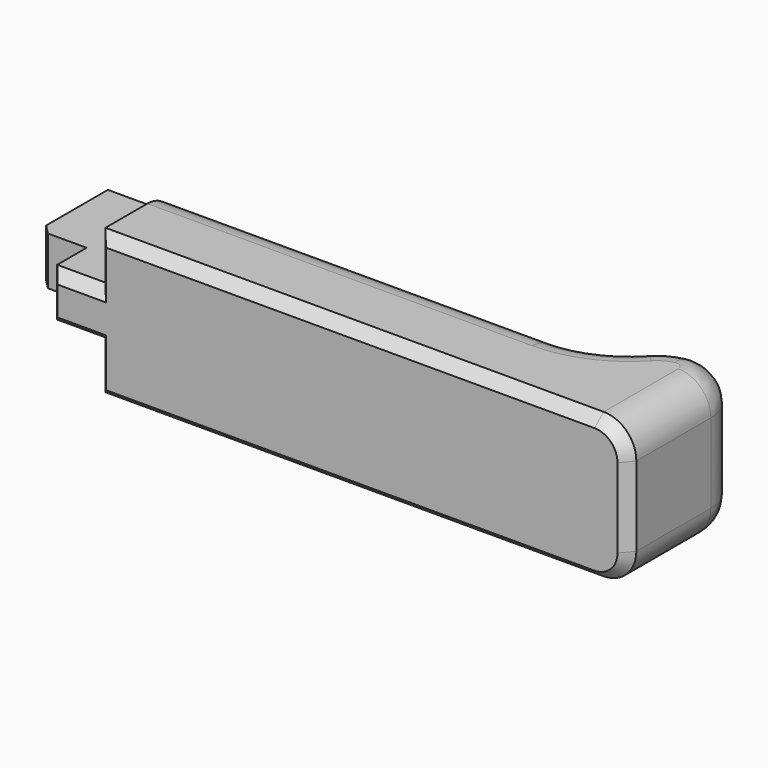
from build123d import *

# Parameters (mm, degrees)
F1_DEPTH    = 5
F0_W        = 20
F0_H        = 10
F2_DEPTH    = 15
F3_T1_DEPTH = 94.3357388745
F4_R        = 8.2083261121
F5_R        = 18.3871550461
F6_R        = 6.7597979746
F7_SIZE2    = 2.3835071852
F7_SIZE     = 2
F8_SIZE     = 2


# Not quite as in the source:
# - a fillet or chamfer that OpenCascade refuses, or shapes differently, is made with other operations: its cross-section is extruded or revolved along the edge and cut away or added


with BuildPart() as f1:
    # F0 (on Top) → F1 (new body, symmetric)
    with BuildSketch(Plane.XY):
        Polygon((-58.0911615491, 10), (-58.0911615491, 0), (-48.0911615491, 0), (-48.0911615491, 20), (-60.0911615491, 20), (-60.0911615491, 30), (-68.0911615491, 30), (-68.0911615491, 10), align=None)
    extrude(amount=F1_DEPTH, both=True)

    # F0 (on Top) → F2 (join, symmetric)
    with BuildSketch(Plane.XY):
        Polygon((-48.0911615491, 20), (-48.0911615491, 0), (61.9088384509, 0), (61.9088384509, 20), (41.9088384509, 20), align=None)
        with Locations((51.9088384509, 25)):
            Rectangle(F0_W, F0_H)
    extrude(amount=F2_DEPTH, both=True)

    # F3: fillet of radius 13.2781745931 on 1 edges, made by hand

    # F3_s2 → F3_t1 (cut)
    with BuildSketch(Plane.XY.offset(-47.1678694372)):
        with BuildLine():
            ThreePointArc((41.9088384509, 20), (46.6279267657, 27.2060539221), (54.7759862258, 30))
            Line((54.7759862258, 30), (41.9088384509, 30))
            Line((41.9088384509, 30), (41.9088384509, 20))
        make_face()
    extrude(amount=F3_T1_DEPTH, mode=Mode.SUBTRACT)

    # F4
    f4_edges = [f1.edges().sort_by_distance(p)[0] for p in [
        (61.908838, 30, 0),
    ]]
    fillet(f4_edges, radius=F4_R)

    # F5
    f5_edges = [f1.edges().sort_by_distance(p)[0] for p in [
        (41.908838, 20, 0),
    ]]
    fillet(f5_edges, radius=F5_R)

    # F6
    f6_edges = [f1.edges().sort_by_distance(p)[0] for p in [
        (-8.204304, 20, -15),
        (-8.204304, 20, 15),
        (48.22996, 28.274291, -15),
        (38.989023, 21.514011, -15),
        (58.852401, 28.06649, -15),
        (61.908838, 10.838145, -15),
        (48.22996, 28.274291, 15),
        (38.989023, 21.514011, 15),
        (58.852401, 28.06649, 15),
        (61.908838, 10.838145, 15),
    ]]
    fillet(f6_edges, radius=F6_R)

    # F7
    f7_edges = [f1.edges().sort_by_distance(p)[0] for p in [
        (3.528939, 0, -15),
        (3.528939, 0, 15),
        (59.928939, 0, 13.020101),
        (61.908838, 0, 0),
        (59.928939, 0, -13.020101),
        (-48.091162, 0, 10),
        (-48.091162, 0, -10),
        (-53.091162, 0, -5),
        (-58.091162, 0, 0),
        (-53.091162, 0, 5),
    ]]
    f7_side = f1.faces().sort_by_distance((4.823554, 0, 0))[0]
    chamfer(f7_edges, length=F7_SIZE, length2=F7_SIZE2, reference=f7_side)

    # F8
    f8_edges = [f1.edges().sort_by_distance(p)[0] for p in [
        (-68.091162, 30, 0),
        (-64.091162, 30, -5),
        (-64.091162, 30, 5),
        (-68.091162, 10, 0),
    ]]
    chamfer(f8_edges, length=F8_SIZE)


solid = f1.part
